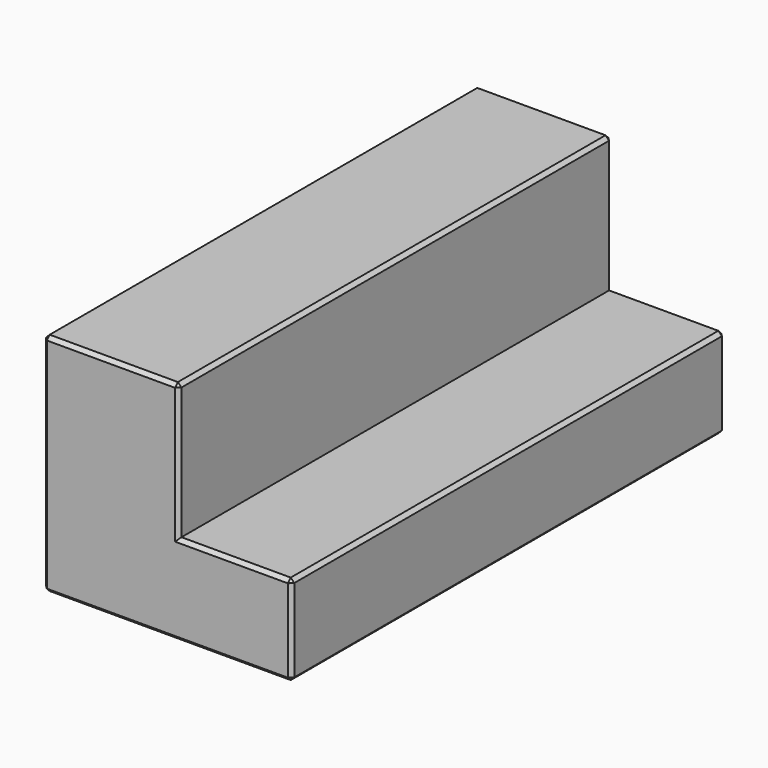
from build123d import *

# Parameters (mm, degrees)
F1_DEPTH = 152.4
F3_SIZE  = 1.016


with BuildPart() as f1:
    # F0 (on Front) → F1 (new body)
    with BuildSketch(Plane.XZ):
        Polygon((0, 63.5), (0, 0), (69.85, 0), (69.85, 25.4), (38.1, 25.4), (38.1, 63.5), align=None)
    extrude(amount=F1_DEPTH)

    # F3
    f3_edges = [f1.edges().sort_by_distance(p)[0] for p in [
        (0, -152.4, 31.75),
        (34.925, -152.4, 0),
        (69.85, -152.4, 12.7),
        (53.975, -152.4, 25.4),
        (38.1, -152.4, 44.45),
        (19.05, -152.4, 63.5),
        (0, 0, 31.75),
        (34.925, 0, 0),
        (69.85, 0, 12.7),
        (53.975, 0, 25.4),
        (38.1, 0, 44.45),
        (19.05, 0, 63.5),
        (38.1, -76.2, 63.5),
        (0, -76.2, 63.5),
        (69.85, -76.2, 0),
        (69.85, -76.2, 25.4),
        (0, -76.2, 0),
    ]]
    chamfer(f3_edges, length=F3_SIZE)


solid = f1.part
